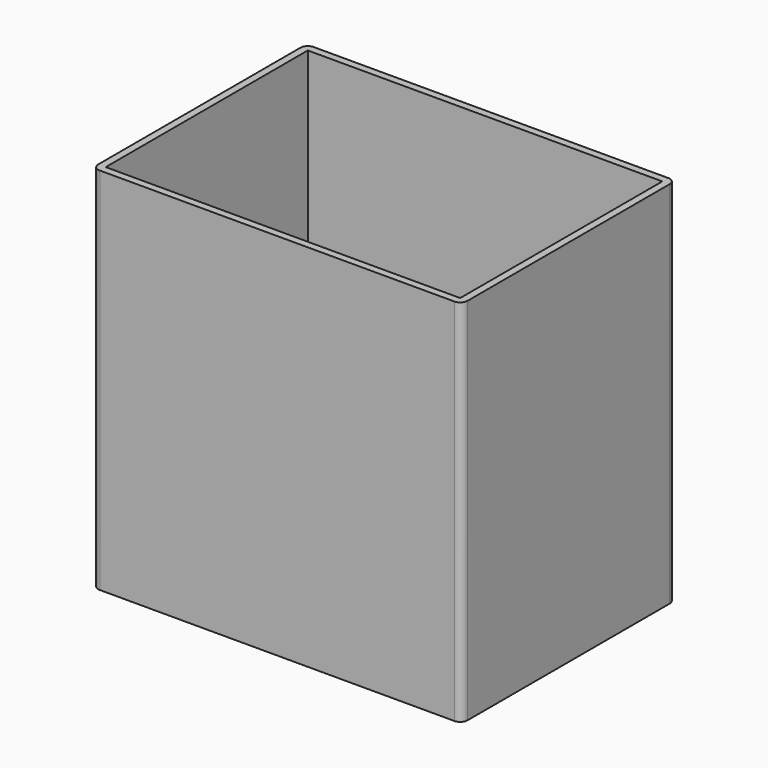
from build123d import *

# Parameters (mm, degrees)
F0_W     = 127
F0_H     = 127
F1_DEPTH = 45.974
F2_R     = 2.54
F3_T     = 2.54


# Not quite as in the source:
# - a shell that OpenCascade refuses in one call is made with other operations: the cavity is built on its own and cut out


with BuildPart() as f1:
    # F0 (on Front) → F1 (new body, symmetric)
    with BuildSketch(Plane.XZ):
        with Locations((-0.4519568912, 63.5)):
            Rectangle(F0_W, F0_H)
    extrude(amount=F1_DEPTH, both=True)

    # F2
    f2_edges = [f1.edges().sort_by_distance(p)[0] for p in [
        (-63.951957, -45.974, 63.5),
        (63.048043, -45.974, 63.5),
        (63.048043, 45.974, 63.5),
        (-63.951957, 45.974, 63.5),
    ]]
    fillet(f2_edges, radius=F2_R)

    # F3: shell of thickness 2.54, made by hand


with BuildPart() as f3_core1:
    # F3_t2: copy of F1
    add(f1.part)

    # the walls: a layer under each face that stays
    f3_faces = [f3_core1.faces().sort_by_distance(p)[0] for p in [
        (-0.4519568912, 45.974, 63.5),
        (63.0480431088, 0, 63.5),
        (-63.9519568912, 0, 63.5),
        (-0.4519568912, -45.974, 63.5),
        (-0.4519568912, 0, 0),
    ]]
    thicken(f3_faces, amount=-F3_T, mode=Mode.SUBTRACT)


with BuildPart() as f1_1:
    add(f1.part)

    # what is left inside the walls is the cavity
    f3_cavity = [f3_core1.part.solids().sort_by_distance(p)[0] for p in [
        (-0.451957, -43.4086, 44.026667),
    ]]
    add(f3_cavity, mode=Mode.SUBTRACT)


solid = f1_1.part
